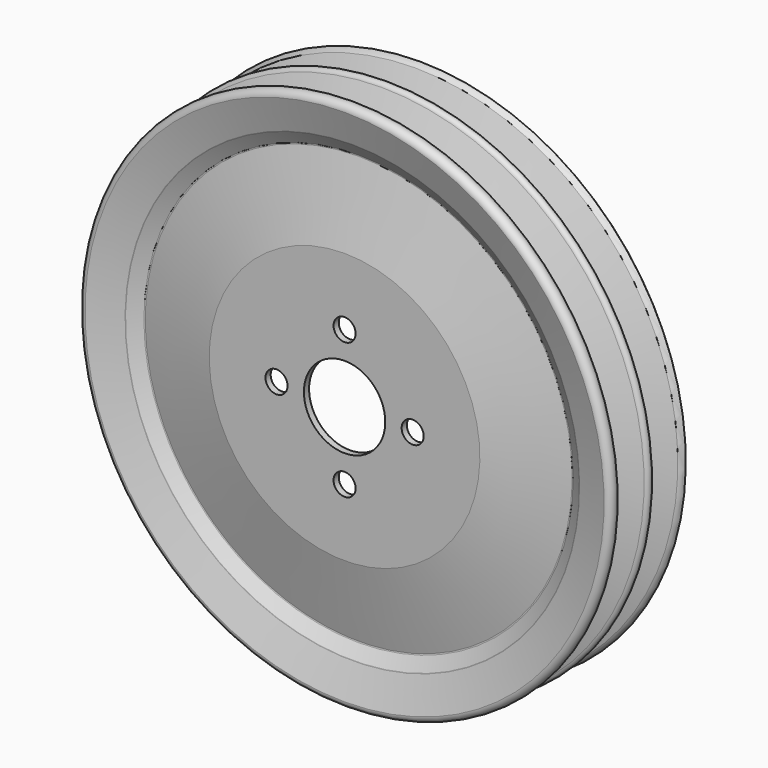
from build123d import *

# Parameters (mm, degrees)
F2_R     = 3.4
F3_DEPTH = 30.001


# Not quite as in the source:
# - ends of sketch curves that miss each other by under 0.0002 mm in the source are joined


with BuildPart() as f1:
    # F0 (on Right) → F1 (revolve)
    with BuildSketch(Plane.YZ):
        with BuildLine():
            Line((0, 12.55), (2, 12.55))
            Line((2, 12.55), (2, 41.741489))
            Line((2, 41.741489), (7.549858, 66.270359))
            ThreePointArc((7.549858, 66.270359), (7.5551419421, 66.4643258691), (7.4861843205, 66.6456982003))
            Line((7.4861843205, 66.6456982003), (4.874038, 70.825131))
            ThreePointArc((4.874038, 70.825131), (4.8425235465, 70.8839575446), (4.8191238849, 70.9464569655))
            Line((4.8191238849, 70.9464569655), (2.249535, 79.511754))
            Line((2.249535, 79.511754), (5.857626, 69.598605))
            ThreePointArc((5.857626, 69.598605), (9, 67.35), (12.1423737717, 69.5986050779))
            Line((12.1423737717, 69.5986050779), (15.454301, 78.698051))
            ThreePointArc((15.454301, 78.698051), (15.5, 78.730049), (15.5456982162, 78.6980507147))
            Line((15.5456982162, 78.6980507147), (18.857626, 69.598605))
            ThreePointArc((18.857626, 69.598605), (22, 67.35), (25.1423737717, 69.5986050779))
            Line((25.1423737717, 69.5986050779), (28.342915, 78.39202))
            ThreePointArc((28.342915, 78.39202), (28.7090314554, 78.8691519685), (29.282608, 79.05))
            Line((29.282608, 79.05), (30, 79.05))
            Line((30, 79.05), (30, 81.05))
            Line((30, 81.05), (29, 82.05))
            ThreePointArc((29, 82.05), (27.9902948071, 81.733069934), (27.1819847697, 81.0500001826))
            Line((27.1819847697, 81.0500001826), (23.254398, 70.259044))
            ThreePointArc((23.254398, 70.259044), (22, 69.35), (20.7456017035, 70.2590439029))
            Line((20.7456017035, 70.2590439029), (16.818015, 81.05))
            ThreePointArc((16.818015, 81.05), (15.5, 82.05), (14.1819848382, 81.0500000452))
            Line((14.1819848382, 81.0500000452), (10.254398, 70.259044))
            ThreePointArc((10.254398, 70.259044), (9, 69.35), (7.7456017035, 70.2590439029))
            Line((7.7456017035, 70.2590439029), (4, 80.55))
            ThreePointArc((4, 80.55), (1.7831758422, 82.0345915451), (-7.457e-07, 80.0500000131))
            Line((-7.457e-07, 80.0500000131), (2.980694, 70.114352))
            ThreePointArc((2.980694, 70.114352), (3.0040933717, 70.0518529309), (3.0356076795, 69.9930267997))
            Line((3.0356076795, 69.9930267997), (5.390899, 66.224562))
            ThreePointArc((5.390899, 66.224562), (5.459855968, 66.0431897166), (5.454572175, 65.8492231867))
            Line((5.454572175, 65.8492231867), (0, 41.741489))
            Line((0, 41.741489), (0, 12.55))
        make_face()
    revolve(axis=Axis((0, 15, 0), (0, 1, 0)))

    # F2 (on Front) → F3 (cut, through all)
    with BuildSketch(Plane.XZ):
        with Locations((0, 21)):
            Circle(F2_R)
        with Locations((21, 0)):
            Circle(F2_R)
        with Locations((0, -21)):
            Circle(F2_R)
        with Locations((-21, 0)):
            Circle(F2_R)
    extrude(amount=-F3_DEPTH, mode=Mode.SUBTRACT)


solid = f1.part
